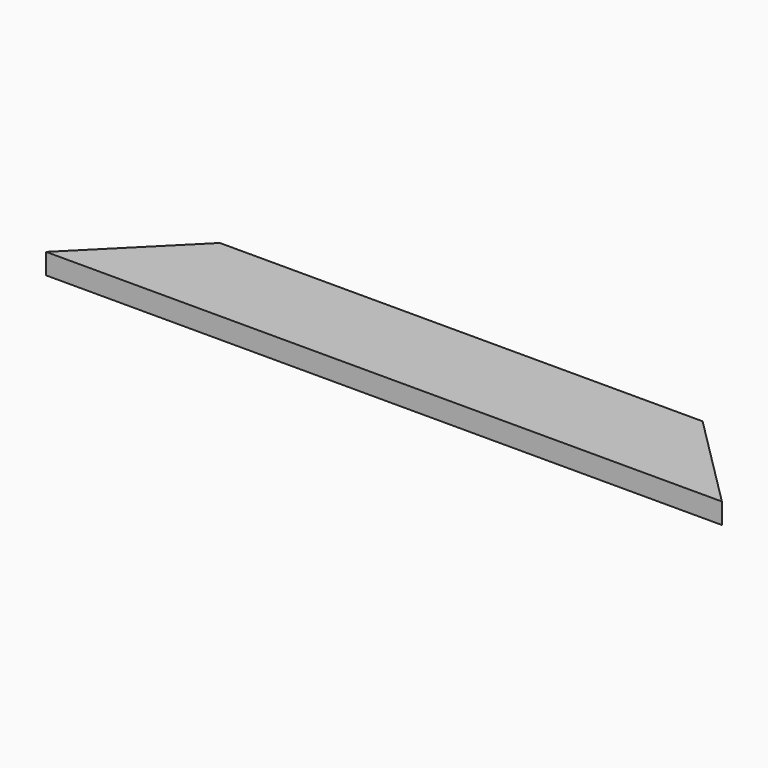
from build123d import *

# Parameters (mm, degrees)
F0_W     = 622.3
F0_H     = 88.9
F1_DEPTH = 19.05
F2_SIZE  = 88.89999
F3_SIZE  = 88.89999


# Not quite as in the source:
# - a fillet or chamfer is up to 0.001 mm smaller than in the source, because OpenCascade refuses the exact size


with BuildPart() as f1:
    # F0 (on Top) → F1 (new body)
    with BuildSketch(Plane.XY):
        with Locations((-221.6517408729, -17.6658927679)):
            Rectangle(F0_W, F0_H)
    extrude(amount=F1_DEPTH)

    # F2 (size 88.9 in the source; OpenCascade refuses exactly that, so slightly less here)
    f2_edges = [f1.edges().sort_by_distance(p)[0] for p in [
        (-532.801741, 26.784107, 9.525),
    ]]
    chamfer(f2_edges, length=F2_SIZE)

    # F3 (size 88.9 in the source; OpenCascade refuses exactly that, so slightly less here)
    f3_edges = [f1.edges().sort_by_distance(p)[0] for p in [
        (89.498259, 26.784107, 9.525),
    ]]
    chamfer(f3_edges, length=F3_SIZE)


solid = f1.part
